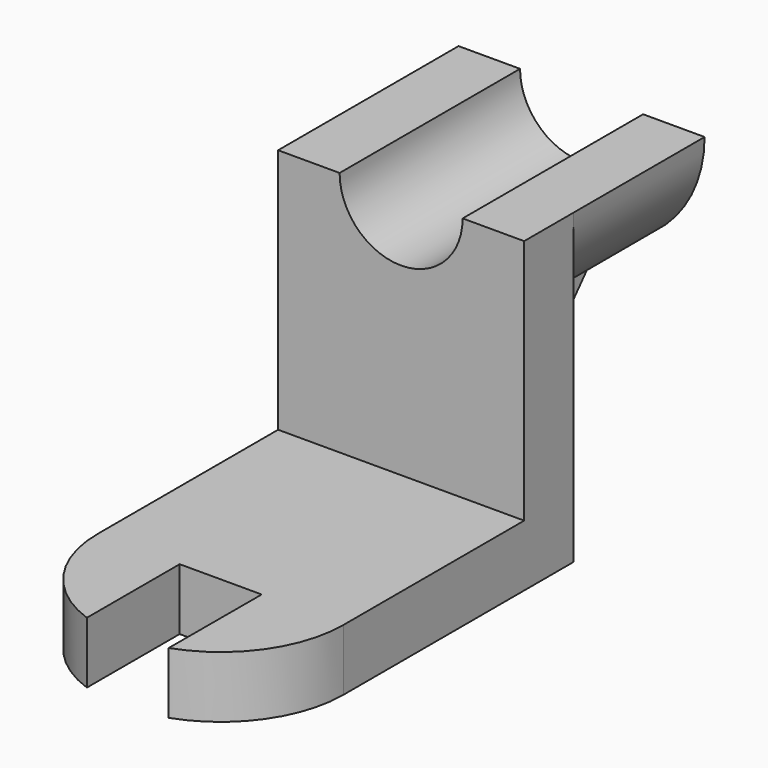
from build123d import *

# Parameters (mm, degrees)
F0_W      = 60
F0_H      = 15
F1_DEPTH  = 75
F2_DEPTH  = 15
F4_DEPTH  = 41.2
F6_DEPTH  = 40
F7_R      = 15
F8_DEPTH  = 168.2
F10_DEPTH = 40
F12_DEPTH = 25


with BuildPart() as f1:
    # F0 (on Top) → F1 (new body)
    with BuildSketch(Plane.XY):
        with Locations((-9.9545444548, 18.6863616109)):
            Rectangle(F0_W, F0_H)
    extrude(amount=F1_DEPTH)

    # F0 (on Top) → F2 (join)
    with BuildSketch(Plane.XY):
        with BuildLine():
            Line((20.0454555452, 11.1863616109), (-39.9545444548, 11.1863616109))
            Line((-39.9545444548, 11.1863616109), (-39.9545444548, -43.8136383891))
            ThreePointArc((-39.9545444548, -43.8136383891), (-9.9545444548, -13.8136383891), (20.0454555452, -43.8136383891))
            Line((20.0454555452, -43.8136383891), (20.0454555452, 11.1863616109))
        make_face()
        with BuildLine():
            ThreePointArc((20.0454555452, -43.8136383891), (-9.9545444548, -13.8136383891), (-39.9545444548, -43.8136383891))
            Line((-39.9545444548, -43.8136383891), (-19.9545444548, -43.8136383891))
            Line((-19.9545444548, -43.8136383891), (-9.9545444548, -43.8136383891))
            Line((-9.9545444548, -43.8136383891), (0.0454555452, -43.8136383891))
            Line((0.0454555452, -43.8136383891), (20.0454555452, -43.8136383891))
        make_face()
        with BuildLine():
            Line((-19.9545444548, -43.8136383891), (-39.9545444548, -43.8136383891))
            ThreePointArc((-39.9545444548, -43.8136383891), (-34.4494418826, -61.1341464648), (-19.9545444548, -72.0979096366))
            Line((-19.9545444548, -72.0979096366), (-19.9545444548, -43.8136383891))
        make_face()
        with BuildLine():
            ThreePointArc((0, -72.1139395306), (14.5264311553, -61.1538181223), (20.0454555452, -43.8136383891))
            Line((20.0454555452, -43.8136383891), (0.0454555452, -43.8136383891))
            Line((0.0454555452, -43.8136383891), (0, -72.1139395306))
        make_face()
        with BuildLine():
            Line((-9.9545444548, -43.8136383891), (-19.9545444548, -43.8136383891))
            Line((-19.9545444548, -43.8136383891), (-19.9545444548, -72.0979096366))
            ThreePointArc((-19.9545444548, -72.0979096366), (-9.9786440611, -73.8136287093), (0, -72.1139395306))
            Line((0, -72.1139395306), (0.0454555452, -43.8136383891))
            Line((0.0454555452, -43.8136383891), (-9.9545444548, -43.8136383891))
        make_face()
    extrude(amount=F2_DEPTH)

    # F3 (on face) → F4 (cut)
    with BuildSketch(Plane.XY.offset(15)):
        with BuildLine():
            Line((-19.9545444548, -43.8136383891), (-19.9545444548, -72.0979096366))
            ThreePointArc((-19.9545444548, -72.0979096366), (-9.9786440611, -73.8136287093), (0, -72.1139395306))
            Line((0, -72.1139395306), (0.0454555452, -43.8136383891))
            Line((0.0454555452, -43.8136383891), (-19.9545444548, -43.8136383891))
        make_face()
    extrude(amount=-F4_DEPTH, mode=Mode.SUBTRACT)

    # F5 (on face) → F6 (join)
    with BuildSketch(Plane(origin=(0, 26.1863616109, 0), x_dir=(-1, 0, 0), z_dir=(0, 1, 0))):
        with BuildLine():
            Line((24.9545444548, 75), (-5.0454555452, 75))
            ThreePointArc((-5.0454555452, 75), (9.9545444548, 60), (24.9545444548, 75))
        make_face()
        with BuildLine():
            ThreePointArc((24.9545444548, 75), (9.9545444548, 60), (-5.0454555452, 75))
            Line((-5.0454555452, 75), (-20.0454555452, 75))
            ThreePointArc((-20.0454555452, 75), (9.9545444548, 45), (39.9545444548, 75))
            Line((39.9545444548, 75), (24.9545444548, 75))
        make_face()
    extrude(amount=F6_DEPTH)

    # F7 (on face) → F8 (cut)
    with BuildSketch(Plane(origin=(0, 66.1863616109, 0), x_dir=(-1, 0, 0), z_dir=(0, 1, 0))):
        with Locations((9.9545444548, 75)):
            Circle(F7_R)
    extrude(amount=-F8_DEPTH, mode=Mode.SUBTRACT)


with BuildPart() as f10:
    # F9 (on face) → F10 (new body)
    with BuildSketch(Plane(origin=(0, 26.1863616109, 0), x_dir=(-1, 0, 0), z_dir=(0, 1, 0))):
        Polygon((14.9545444548, 45.4196010845), (4.9545444548, 0), (14.9545444548, 0), align=None)
        with BuildLine():
            Line((4.9545444548, 45.4196010845), (4.9545444548, 0))
            Line((4.9545444548, 0), (14.9545444548, 45.4196010845))
            ThreePointArc((14.9545444548, 45.4196010845), (9.9545444548, 45), (4.9545444548, 45.4196010845))
        make_face()
    extrude(amount=F10_DEPTH)


with BuildPart() as f12_tool:
    # F11 (on face) → F12 (new body)
    with BuildSketch(Plane.YZ.offset(-4.9545444548)):
        Polygon((66.1863616109, 0), (66.1863616109, 45.4196010845), (26.1863616109, 0), align=None)
    extrude(amount=-F12_DEPTH)


with BuildPart() as f1_1:
    add(f1.part)

    # F12: cut by f12_tool
    add(f12_tool.part, mode=Mode.SUBTRACT)


with BuildPart() as f10_1:
    add(f10.part)

    # F12: cut by f12_tool
    add(f12_tool.part, mode=Mode.SUBTRACT)


solid = Compound([f1_1.part, f10_1.part])
